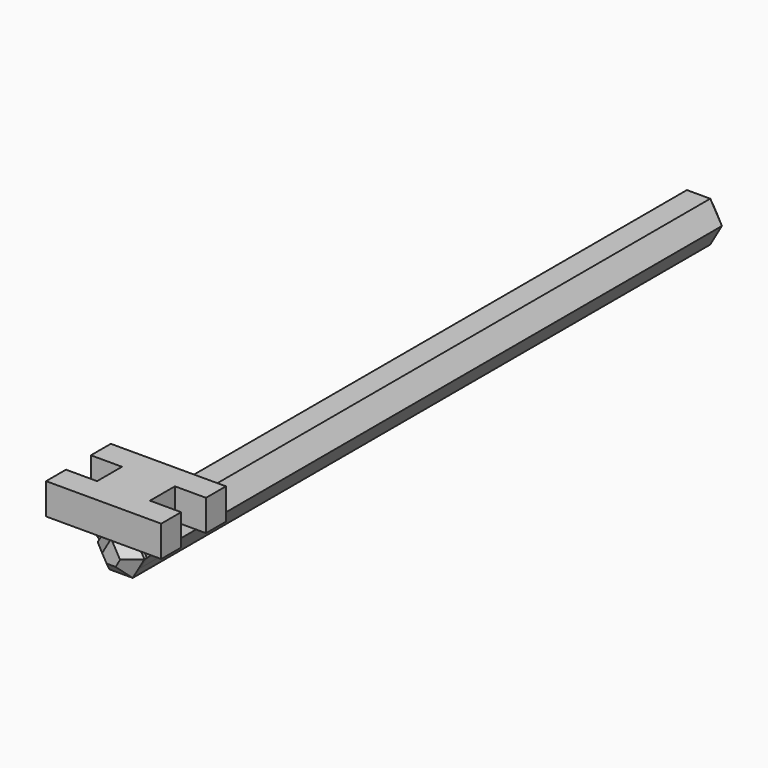
from build123d import *

# Parameters (mm, degrees)
F1_DEPTH      = 60
F2_W          = 2.3736116251
F2_H          = 5
F2_W_2        = 3.7527767497
F3_DEPTH      = 5
F5_DEPTH      = 4
F7_DEPTH      = 4
F8_W          = 4
F8_H          = 5
F9_DEPTH      = 5
F10_W         = 4
F10_H         = 5
F11_DEPTH     = 5
F12_T4_DEPTH  = 16.3154051471
F12_T9_DEPTH  = 16.3154051471
F13_T1_DEPTH  = 14.0395087016
F13_T3_DEPTH  = 14.0395087016
F13_T5_DEPTH  = 14.0395087016
F13_T7_DEPTH  = 14.0395087016
F13_T9_DEPTH  = 14.0395087016
F13_T14_DEPTH = 14.0395087016
F13_T19_DEPTH = 14.0395087016
F13_T24_DEPTH = 14.0395087016
F13_T29_DEPTH = 14.0395087016


# Not quite as in the source:
# - a fillet or chamfer that OpenCascade refuses, or shapes differently, is made with other operations: its cross-section is extruded or revolved along the edge and cut away or added


with BuildPart() as f1:
    # F0 (on Front) → F1 (new body, symmetric)
    with BuildSketch(Plane.XZ):
        Polygon((1.8763883749, -3.25), (3.7527767497, 0), (1.8763883749, 3.25), (-1.8763883749, 3.25), (-3.7527767497, 0), (-1.8763883749, -3.25), align=None)
    extrude(amount=F1_DEPTH, both=True)

    # F2 (on face) → F3 (join, symmetric)
    with BuildSketch(Plane.XY.offset(3.25)):
        with Locations((-3.0631941874, -55)):
            Rectangle(F2_W, F2_H)
        with Locations((0, -55)):
            Rectangle(F2_W_2, F2_H)
        with Locations((3.0631941874, -55)):
            Rectangle(F2_W, F2_H)
    extrude(amount=F3_DEPTH, both=True)

    # F4 (on face) → F5 (join)
    with BuildSketch(Plane.XZ.offset(57.5)):
        Polygon((-4.25, 8.25), (-4.25, 3.25), (-1.8763883749, 3.25), (1.8763883749, 3.25), (4.25, 3.25), (4.25, 8.25), align=None)
    extrude(amount=F5_DEPTH)

    # F6 (on face) → F7 (join)
    with BuildSketch(Plane(origin=(0, -52.5, 0), x_dir=(-1, 0, 0), z_dir=(0, 1, 0))):
        Polygon((-4.25, 8.25), (-4.25, 3.25), (-1.8763883749, 3.25), (1.8763883749, 3.25), (4.25, 3.25), (4.25, 8.25), align=None)
    extrude(amount=F7_DEPTH)

    # F8 (on face) → F9 (join)
    with BuildSketch(Plane.YZ.offset(4.25)):
        with Locations((-59.5, 5.75)):
            Rectangle(F8_W, F8_H)
        with Locations((-50.5, 5.75)):
            Rectangle(F8_W, F8_H)
    extrude(amount=F9_DEPTH)

    # F10 (on face) → F11 (join)
    with BuildSketch(Plane(origin=(-4.25, 0, 0), x_dir=(0, -1, 0), z_dir=(-1, 0, 0))):
        with Locations((50.5, 5.75)):
            Rectangle(F10_W, F10_H)
        with Locations((59.5, 5.75)):
            Rectangle(F10_W, F10_H)
    extrude(amount=F11_DEPTH)

    # F12: chamfer of 2.2 on 2 edges, made by hand


with BuildPart() as f12_tool2:
    # F12_s3 → F12_t4 (new body)
    with BuildSketch(Plane.XZ.offset(63.1577025735)):
        Polygon((4.25, 0.45), (2.05, -1.75), (4.25, -1.75), align=None)
    extrude(amount=-F12_T4_DEPTH)

    split(bisect_by=Plane(origin=(2.8145825623, 0, -1.625), x_dir=(0, 1, 0), z_dir=(0.8660254038, 0, -0.5)), keep=Keep.TOP)


with BuildPart() as f1_1:
    add(f1.part)

    # F12_t1: cut F12_tool2
    add(f12_tool2.part, mode=Mode.SUBTRACT)


with BuildPart() as f12_tool7:
    # F12_s8 → F12_t9 (new body)
    with BuildSketch(Plane.XZ.offset(46.8422974265)):
        Polygon((-4.25, 0.45), (-2.05, -1.75), (-4.25, -1.75), align=None)
    extrude(amount=F12_T9_DEPTH)

    split(bisect_by=Plane(origin=(-2.8145825623, 0, -1.625), x_dir=(0, 1, 0), z_dir=(-0.8660254038, 0, -0.5)), keep=Keep.TOP)


with BuildPart() as f1_2:
    add(f1_1.part)

    # F12_t6: cut F12_tool7
    add(f12_tool7.part, mode=Mode.SUBTRACT)

    # F13: chamfer of 2 on 11 edges, made by hand

    # F13_s2 → F13_t1 (cut)
    with BuildSketch(Plane(origin=(-3.5098771754, 0, -6.0792855961), x_dir=(0, 1, 0), z_dir=(0.5, 0, 0.8660254038))):
        Polygon((58, -3.25), (60, -1.25), (60, -3.25), align=None)
    extrude(amount=F13_T1_DEPTH, mode=Mode.SUBTRACT)

    # F13_s4 → F13_t3 (cut)
    with BuildSketch(Plane(origin=(3.5098771754, 0, -6.0792855961), x_dir=(0, 1, 0), z_dir=(-0.5, 0, 0.8660254038))):
        Polygon((58, -3.25), (60, -1.25), (60, -3.25), align=None)
    extrude(amount=F13_T3_DEPTH, mode=Mode.SUBTRACT)

    # F13_s6 → F13_t5 (cut)
    with BuildSketch(Plane.YZ.offset(-7.0197543508)):
        Polygon((58, 3.25), (60, 1.25), (60, 3.25), align=None)
        Polygon((60, -1.25), (58, -3.25), (60, -3.25), align=None)
        Polygon((-60, -1.25), (-58, -3.25), (-60, -3.25), align=None)
    extrude(amount=F13_T5_DEPTH, mode=Mode.SUBTRACT)

    # F13_s8 → F13_t7 (cut)
    with BuildSketch(Plane(origin=(3.5098771754, 0, 6.0792855961), x_dir=(0, 1, 0), z_dir=(-0.5, 0, -0.8660254038))):
        Polygon((58, -3.25), (60, -1.25), (60, -3.25), align=None)
    extrude(amount=F13_T7_DEPTH, mode=Mode.SUBTRACT)

    # F13_s10 → F13_t9 (cut)
    with BuildSketch(Plane(origin=(-3.5098771754, 0, 6.0792855961), x_dir=(0, 1, 0), z_dir=(0.5, 0, -0.8660254038))):
        Polygon((58, -3.25), (60, -1.25), (60, -3.25), align=None)
    extrude(amount=F13_T9_DEPTH, mode=Mode.SUBTRACT)


with BuildPart() as f13_tool12:
    # F13_s13 → F13_t14 (new body)
    with BuildSketch(Plane(origin=(-3.5098771754, 0, 6.0792855961), x_dir=(0, 1, 0), z_dir=(0.5, 0, -0.8660254038))):
        Polygon((-60, -1.25), (-58, -3.25), (-60, -3.25), align=None)
    extrude(amount=F13_T14_DEPTH)

    split(bisect_by=Plane.XY.offset(3.25), keep=Keep.BOTTOM)


with BuildPart() as f1_3:
    add(f1_2.part)

    # F13_t11: cut F13_tool12
    add(f13_tool12.part, mode=Mode.SUBTRACT)


with BuildPart() as f13_tool17:
    # F13_s18 → F13_t19 (new body)
    with BuildSketch(Plane(origin=(3.5098771754, 0, 6.0792855961), x_dir=(0, 1, 0), z_dir=(-0.5, 0, -0.8660254038))):
        Polygon((-58, 3.25), (-60, 1.25), (-60, 3.25), align=None)
    extrude(amount=F13_T19_DEPTH)

    split(bisect_by=Plane(origin=(2.8145825623, 0, 1.625), x_dir=(0, 1, 0), z_dir=(-0.8660254038, 0, -0.5)), keep=Keep.TOP)


with BuildPart() as f1_4:
    add(f1_3.part)

    # F13_t16: cut F13_tool17
    add(f13_tool17.part, mode=Mode.SUBTRACT)


with BuildPart() as f13_tool22:
    # F13_s23 → F13_t24 (new body)
    with BuildSketch(Plane(origin=(3.5098771754, 0, -6.0792855961), x_dir=(0, 1, 0), z_dir=(-0.5, 0, 0.8660254038))):
        Polygon((-60, -1.25), (-58, -3.25), (-60, -3.25), align=None)
    extrude(amount=F13_T24_DEPTH)

    split(bisect_by=Plane.XY.offset(3.25), keep=Keep.BOTTOM)


with BuildPart() as f1_5:
    add(f1_4.part)

    # F13_t21: cut F13_tool22
    add(f13_tool22.part, mode=Mode.SUBTRACT)


with BuildPart() as f13_tool27:
    # F13_s28 → F13_t29 (new body)
    with BuildSketch(Plane(origin=(3.5098771754, 0, 6.0792855961), x_dir=(0, 1, 0), z_dir=(-0.5, 0, -0.8660254038))):
        Polygon((-60, -1.25), (-58, -3.25), (-60, -3.25), align=None)
    extrude(amount=F13_T29_DEPTH)

    split(bisect_by=Plane.XY.offset(3.25), keep=Keep.BOTTOM)


with BuildPart() as f1_6:
    add(f1_5.part)

    # F13_t26: cut F13_tool27
    add(f13_tool27.part, mode=Mode.SUBTRACT)


solid = f1_6.part
